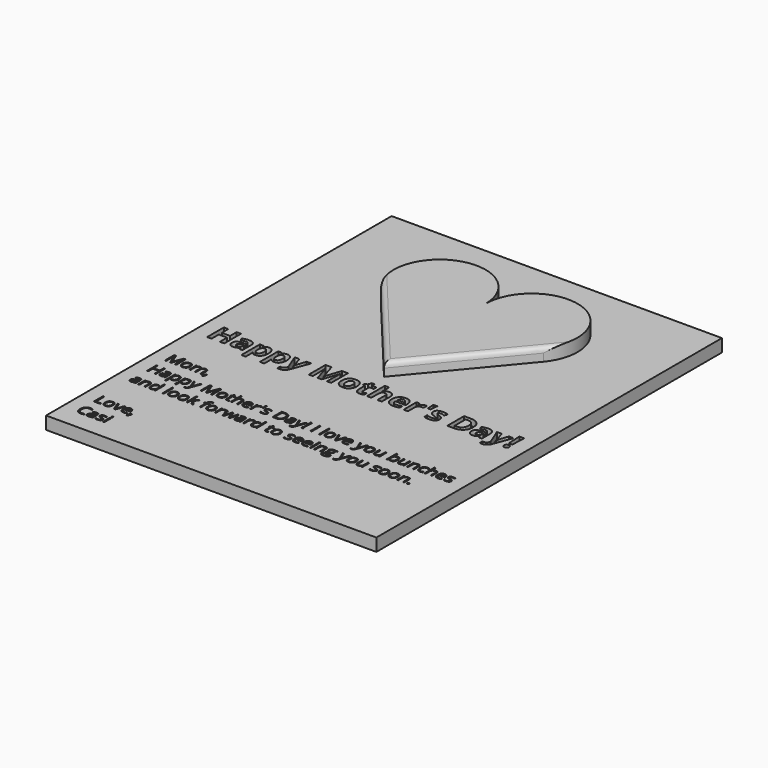
from build123d import *

# Parameters (mm, degrees)
F0_W           = 82.55
F0_H           = 107.95
F1_DEPTH       = 3.175
F3_DEPTH       = 3.175
F4_TEXT_SIZE   = 7.3334235575
F4_TEXT_SIZE_2 = 4.077796545
F5_DEPTH       = 1.5875
F6_T1_DEPTH    = 40.3225
F6_T3_DEPTH    = 40.3225


# Not quite as in the source:
# - a fillet or chamfer that OpenCascade refuses, or shapes differently, is made with other operations: its cross-section is extruded or revolved along the edge and cut away or added
# - Text() gives the source's letters only with a copy of the font that has no kerning and outlines rounded to 1/6400 em; it was checked with that copy


with BuildPart() as f1:
    # F0 (on Top) → F1 (new body)
    with BuildSketch(Plane.XY):
        Rectangle(F0_W, F0_H)
    extrude(amount=F1_DEPTH)

    # F2 (on face) → F3 (join)
    with BuildSketch(Plane.XY.offset(3.175)):
        with BuildLine():
            Line((-20.32, 24.3959033446), (0, 0))
            Line((0, 0), (20.32, 24.3959033446))
            ThreePointArc((20.32, 24.3959033446), (15.4012298635, 42.5549194538), (0, 31.75))
            ThreePointArc((0, 31.75), (-15.4012298635, 42.5549194538), (-20.32, 24.3959033446))
        make_face()
    extrude(amount=F3_DEPTH)

    # F4 (on face) → F5 (cut)
    with BuildSketch(Plane.XY.offset(3.175)):
        with Locations((-38.1, -8.4550649614)):
            Text("Happy Mother's Day!", F4_TEXT_SIZE, font='Open Sans', font_style=FontStyle.BOLD, text_align=(TextAlign.LEFT, TextAlign.BOTTOM))
        with Locations((-38.1, -21.3510135124)):
            Text('Mom,', F4_TEXT_SIZE_2, font='Open Sans', text_align=(TextAlign.LEFT, TextAlign.BOTTOM))
        with Locations((-38.1, -26.8968168136)):
            Text("Happy Mother's Day! I love you bunches", F4_TEXT_SIZE_2, font='Open Sans', text_align=(TextAlign.LEFT, TextAlign.BOTTOM))
        with Locations((-38.1, -32.4426201147)):
            Text('and look forward to seeing you soon.', F4_TEXT_SIZE_2, font='Open Sans', text_align=(TextAlign.LEFT, TextAlign.BOTTOM))
        with Locations((-38.1, -43.5342267171)):
            Text('Love,', F4_TEXT_SIZE_2, font='Open Sans', text_align=(TextAlign.LEFT, TextAlign.BOTTOM))
        with Locations((-38.1, -49.0800300182)):
            Text('Casi', F4_TEXT_SIZE_2, font='Open Sans', text_align=(TextAlign.LEFT, TextAlign.BOTTOM))
    extrude(amount=-F5_DEPTH, mode=Mode.SUBTRACT)

    # F6: fillet of radius 1.27 on 2 edges, made by hand

    # F6_s2 → F6_t1 (cut)
    with BuildSketch(Plane(origin=(-23.7744, 28.5432069132, 0), x_dir=(0, 0, 1), z_dir=(0.64, -0.7683749085, 0))):
        with BuildLine():
            add(Edge.make_bspline(
                [(5.08, 0), (6.35, 0), (6.35, -1.27)],
                knots=[0, 0, 0, 1, 1, 1], degree=2, weights=[1, 1, 1]))
            Line((6.35, -1.27), (6.35, 0))
            Line((6.35, 0), (5.08, 0))
        make_face()
    extrude(amount=F6_T1_DEPTH, mode=Mode.SUBTRACT)

    # F6_s4 → F6_t3 (cut)
    with BuildSketch(Plane(origin=(-2.032, -2.4395903345, 0), x_dir=(0, 0, 1), z_dir=(0.64, 0.7683749085, 0))):
        with BuildLine():
            add(Edge.make_bspline(
                [(5.08, 0), (6.35, 0), (6.35, -1.27)],
                knots=[0, 0, 0, 1, 1, 1], degree=2, weights=[1, 1, 1]))
            Line((6.35, -1.27), (6.35, 0))
            Line((6.35, 0), (5.08, 0))
        make_face()
    extrude(amount=F6_T3_DEPTH, mode=Mode.SUBTRACT)


solid = f1.part
